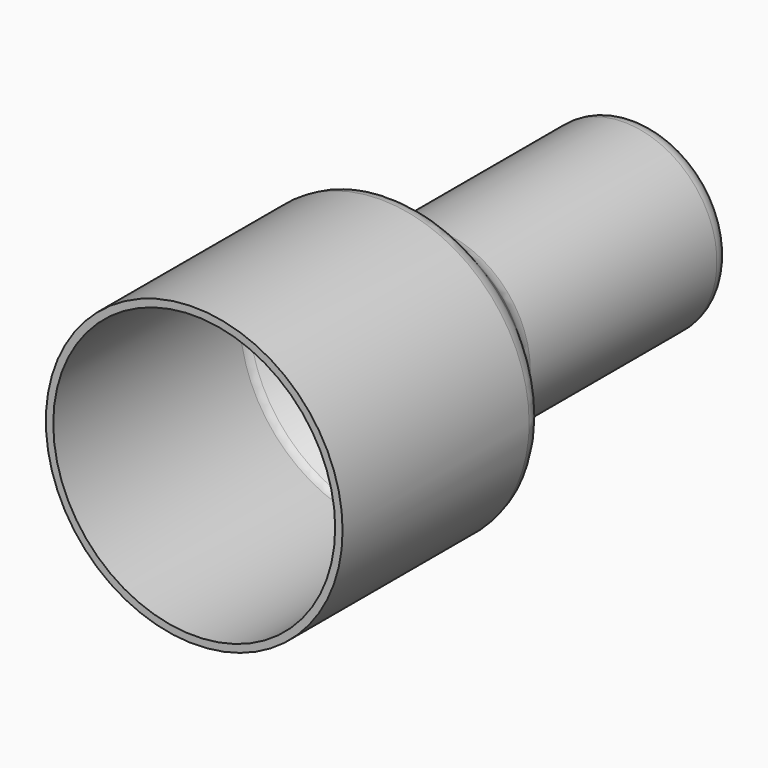
from build123d import *

# Parameters (mm, degrees)
F0_R        = 40.0443714264
F1_DEPTH    = 80
F2_R        = 25.0697968859
F3_DEPTH    = 70
F4_S5_R     = 25.0697968859
F4_T6_DEPTH = 59
F5_R        = 5
F6_R        = 5
F7_T        = -2


# Not quite as in the source:
# - a fillet or chamfer that OpenCascade refuses, or shapes differently, is made with other operations: its cross-section is extruded or revolved along the edge and cut away or added


with BuildPart() as f1:
    # F0 (on Front) → F1 (new body)
    with BuildSketch(Plane.XZ):
        Circle(F0_R)
    extrude(amount=-F1_DEPTH)

    # F2 (on face) → F3 (join)
    with BuildSketch(Plane(origin=(0, 80, 0), x_dir=(-1, 0, 0), z_dir=(0, 1, 0))):
        Circle(F2_R)
    extrude(amount=F3_DEPTH)

    # F4: chamfer of 15 on 1 edges, made by hand


with BuildPart() as f4_tool2:
    # F4_s3 → F4_t4 (revolve)
    with BuildSketch(Plane.XY):
        Polygon((40.0443714264, 65), (25.0443714264, 80), (40.0443714264, 80), align=None)
    revolve(axis=Axis((0, 80, 0), (0, -1, 0)))

    # F4_s5 → F4_t6 (cut, symmetric)
    with BuildSketch(Plane.XZ.offset(-72.5)):
        Circle(F4_S5_R)
    extrude(amount=F4_T6_DEPTH, both=True, mode=Mode.SUBTRACT)


with BuildPart() as f1_1:
    add(f1.part)

    # F4_t1: cut F4_tool2
    add(f4_tool2.part, mode=Mode.SUBTRACT)

    # F5
    f5_edges = [f1_1.edges().sort_by_distance(p)[0] for p in [
        (25.069797, 150, 0),
    ]]
    fillet(f5_edges, radius=F5_R)

    # F6
    f6_edges = [f1_1.edges().sort_by_distance(p)[0] for p in [
        (32.557084, 72.487287, 0),
        (-25.069797, 79.974575, 0),
        (-40.044371, 65, 0),
    ]]
    fillet(f6_edges, radius=F6_R)

    # F7
    f7_openings = [f1_1.faces().sort_by_distance(p)[0] for p in [
        (0, 0, 0),
    ]]
    offset(amount=F7_T, openings=f7_openings)


solid = f1_1.part
